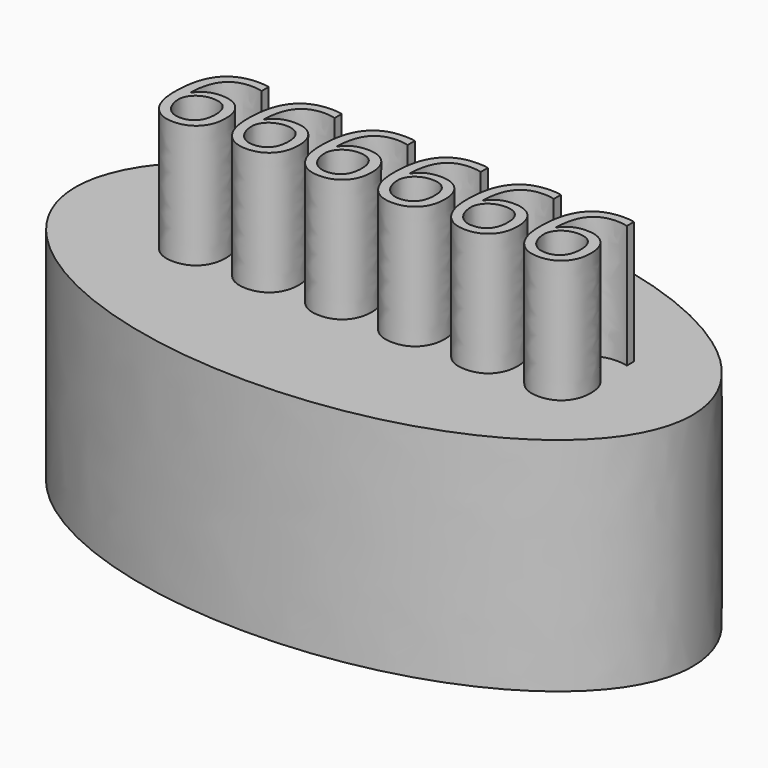
from build123d import *

# Parameters (mm, degrees)
F1_DEPTH     = 45.72
F2_TEXT_SIZE = 26.3902513931
F3_DEPTH     = 25.4


# Not quite as in the source:
# - Text() gives the source's letters only with a copy of the font that has no kerning and outlines rounded to 1/6400 em; it was checked with that copy


with BuildPart() as f1:
    # F0 (on Top) → F1 (new body)
    with BuildSketch(Plane.XY):
        with BuildLine():
            add(Edge.make_bspline(
                [(63.7324601412, 0), (63.7324601412, 61.622520235), (-31.8662300706, 30.8112601175), (-127.4649202824, 0), (-31.8662300706, -30.8112601175), (63.7324601412, -61.622520235), (63.7324601412, 0)],
                knots=[0, 0, 0, 2.0943951024, 2.0943951024, 4.1887902048, 4.1887902048, 6.2831853072, 6.2831853072, 6.2831853072], degree=2, weights=[1, 0.5, 1, 0.5, 1, 0.5, 1]))
        make_face()
    extrude(amount=F1_DEPTH)


with BuildPart() as f3:
    # F2 (on face) → F3 (new body)
    with BuildSketch(Plane.XY.offset(45.72)):
        with Locations((-43.1208759546, -10.168123059)):
            Text('666666', F2_TEXT_SIZE, font='Open Sans', text_align=(TextAlign.LEFT, TextAlign.BOTTOM))
    extrude(amount=F3_DEPTH)


solid = Compound([f1.part, f3.part])
